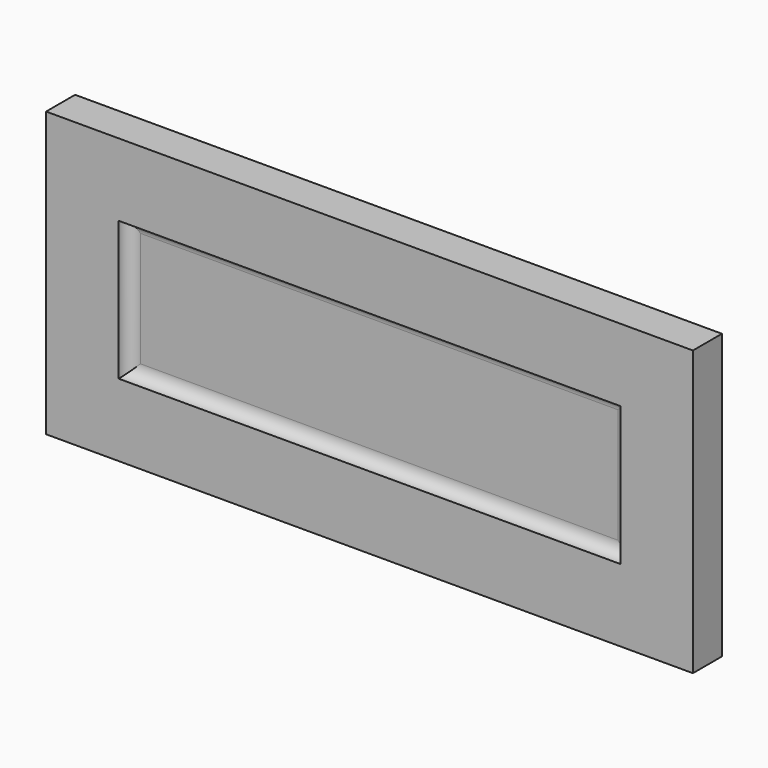
from build123d import *

# Parameters (mm, degrees)
F0_W     = 339.725
F0_H     = 149.225
F0_W_2   = 263.525
F0_H_2   = 73.025
F1_DEPTH = 19.05
F2_DEPTH = 12.7
F3_R     = 6.34999


# Not quite as in the source:
# - a fillet or chamfer is up to 0.001 mm smaller than in the source, because OpenCascade refuses the exact size


with BuildPart() as f1:
    # F0 (on Front) → F1 (new body)
    with BuildSketch(Plane.XZ):
        Rectangle(F0_W, F0_H)
        Rectangle(F0_W_2, F0_H_2, mode=Mode.SUBTRACT)
    extrude(amount=F1_DEPTH)

    # F0 (on Front) → F2 (join)
    with BuildSketch(Plane.XZ):
        Rectangle(F0_W_2, F0_H_2)
    extrude(amount=F2_DEPTH)

    # F3 (radius 6.35 in the source; OpenCascade refuses exactly that, so slightly less here)
    f3_edges = [f1.edges().sort_by_distance(p)[0] for p in [
        (0, -12.7, 36.5125),
        (-131.7625, -12.7, 0),
        (0, -12.7, -36.5125),
        (131.7625, -12.7, 0),
    ]]
    fillet(f3_edges, radius=F3_R)


solid = f1.part
